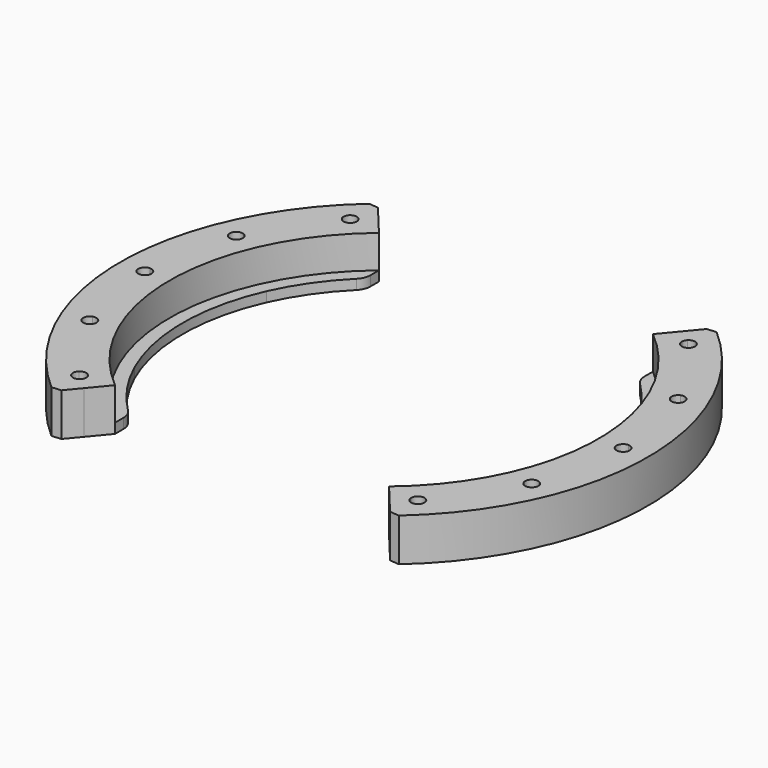
from build123d import *

# Parameters (mm, degrees)
F1_DEPTH    = 3
F2_DEPTH    = 13
F3_R        = 5
F4_T1_DEPTH = 23.5438904605


# Not quite as in the source:
# - a fillet or chamfer that OpenCascade refuses, or shapes differently, is made with other operations: its cross-section is extruded or revolved along the edge and cut away or added


with BuildPart() as f1:
    # F0 (on Top) → F1 (new body)
    with BuildSketch(Plane.XY):
        with BuildLine():
            ThreePointArc((-55.641710973, -25), (-61, 0), (-55.641710973, 25))
            ThreePointArc((-55.641710973, 25), (-49.5734728737, 35.5453342541), (-41.5331193146, 44.6766158074))
            Line((-41.5331193146, 44.6766158074), (-41.5331193146, 50))
            ThreePointArc((-41.5331193146, 50), (-65, 0), (-41.5331193146, -50))
            Line((-41.5331193146, -50), (-41.5331193146, -44.6766158074))
            ThreePointArc((-41.5331193146, -44.6766158074), (-49.5734728737, -35.5453342541), (-55.641710973, -25))
        make_face()
    extrude(amount=F1_DEPTH)



with BuildPart() as f1b:
    # F0 (on Top) → F1, piece 2 (new body)
    with BuildSketch(Plane.XY):
        with BuildLine():
            ThreePointArc((-49.8316562129, 52.6598142712), (-48.1036598795, 54.2428604168), (-46.3254023124, 55.7692307692))
            Line((-46.3254023124, 55.7692307692), (-51.1176853103, 61.5384615385))
            ThreePointArc((-51.1176853103, 61.5384615385), (-80, 0), (-51.1176853103, -61.5384615385))
            Line((-51.1176853103, -61.5384615385), (-46.3254023124, -55.7692307692))
            ThreePointArc((-46.3254023124, -55.7692307692), (-48.1036598795, -54.2428604168), (-49.8316562129, -52.6598142712))
            ThreePointArc((-49.8316562129, -52.6598142712), (-52.6794551984, -52.6794551984), (-52.6598142712, -49.8316562129))
            ThreePointArc((-52.6598142712, -49.8316562129), (-60.2815468919, -40.2788418939), (-66.1904857193, -29.581575351))
            ThreePointArc((-66.1904857193, -29.581575351), (-68.8290251721, -28.5099157112), (-67.721073831, -25.8864087733))
            ThreePointArc((-67.721073831, -25.8864087733), (-71.1069328292, -14.1440483462), (-72.4724137931, -1.9998097412))
            ThreePointArc((-72.4724137931, -1.9998097412), (-74.5, 0), (-72.4724137931, 1.9998097412))
            ThreePointArc((-72.4724137931, 1.9998097412), (-71.1069328292, 14.1440483462), (-67.721073831, 25.8864087733))
            ThreePointArc((-67.721073831, 25.8864087733), (-68.8290251721, 28.5099157112), (-66.1904857193, 29.581575351))
            ThreePointArc((-66.1904857193, 29.581575351), (-60.2815468919, 40.2788418939), (-52.6598142712, 49.8316562129))
            ThreePointArc((-52.6598142712, 49.8316562129), (-52.6794551984, 52.6794551984), (-49.8316562129, 52.6598142712))
        make_face()
    extrude(amount=F1_DEPTH)


with BuildPart() as f1_1:
    add(f1.part)

    add(f1b.part)  # F2 merges F1b
    # F0 (on Top) → F2 (join)
    with BuildSketch(Plane.XY):
        with BuildLine():
            ThreePointArc((-41.5331193146, -50), (-65, 0), (-41.5331193146, 50))
            Line((-41.5331193146, 50), (-46.3254023124, 55.7692307692))
            ThreePointArc((-46.3254023124, 55.7692307692), (-48.1036598795, 54.2428604168), (-49.8316562129, 52.6598142712))
            ThreePointArc((-49.8316562129, 52.6598142712), (-49.4122479979, 52.0178468293), (-49.265241636, 51.265241636))
            ThreePointArc((-49.265241636, 51.265241636), (-50.4871495047, 49.4228050333), (-52.6598142712, 49.8316562129))
            ThreePointArc((-52.6598142712, 49.8316562129), (-60.2815468919, 40.2788418939), (-66.1904857193, 29.581575351))
            ThreePointArc((-66.1904857193, 29.581575351), (-65.3107032116, 28.8441940675), (-64.9812661071, 27.7445488465))
            ThreePointArc((-64.9812661071, 27.7445488465), (-65.8586832477, 26.0893123909), (-67.721073831, 25.8864087733))
            ThreePointArc((-67.721073831, 25.8864087733), (-71.1069328292, 14.1440483462), (-72.4724137931, 1.9998097412))
            ThreePointArc((-72.4724137931, 1.9998097412), (-71.0760666424, 1.4044264997), (-70.5, 0))
            ThreePointArc((-70.5, 0), (-71.0760666424, -1.4044264997), (-72.4724137931, -1.9998097412))
            ThreePointArc((-72.4724137931, -1.9998097412), (-71.1069328292, -14.1440483462), (-67.721073831, -25.8864087733))
            ThreePointArc((-67.721073831, -25.8864087733), (-65.8586832477, -26.0893123909), (-64.9812661071, -27.7445488465))
            ThreePointArc((-64.9812661071, -27.7445488465), (-65.3107032116, -28.8441940675), (-66.1904857193, -29.581575351))
            ThreePointArc((-66.1904857193, -29.581575351), (-60.2815468919, -40.2788418939), (-52.6598142712, -49.8316562129))
            ThreePointArc((-52.6598142712, -49.8316562129), (-50.4871495047, -49.4228050333), (-49.265241636, -51.265241636))
            ThreePointArc((-49.265241636, -51.265241636), (-49.4122479979, -52.0178468293), (-49.8316562129, -52.6598142712))
            ThreePointArc((-49.8316562129, -52.6598142712), (-48.1036598795, -54.2428604168), (-46.3254023124, -55.7692307692))
            Line((-46.3254023124, -55.7692307692), (-41.5331193146, -50))
        make_face()
        with BuildLine():
            ThreePointArc((-49.8316562129, 52.6598142712), (-48.1036598795, 54.2428604168), (-46.3254023124, 55.7692307692))
            Line((-46.3254023124, 55.7692307692), (-51.1176853103, 61.5384615385))
            ThreePointArc((-51.1176853103, 61.5384615385), (-80, 0), (-51.1176853103, -61.5384615385))
            Line((-51.1176853103, -61.5384615385), (-46.3254023124, -55.7692307692))
            ThreePointArc((-46.3254023124, -55.7692307692), (-48.1036598795, -54.2428604168), (-49.8316562129, -52.6598142712))
            ThreePointArc((-49.8316562129, -52.6598142712), (-52.6794551984, -52.6794551984), (-52.6598142712, -49.8316562129))
            ThreePointArc((-52.6598142712, -49.8316562129), (-60.2815468919, -40.2788418939), (-66.1904857193, -29.581575351))
            ThreePointArc((-66.1904857193, -29.581575351), (-68.8290251721, -28.5099157112), (-67.721073831, -25.8864087733))
            ThreePointArc((-67.721073831, -25.8864087733), (-71.1069328292, -14.1440483462), (-72.4724137931, -1.9998097412))
            ThreePointArc((-72.4724137931, -1.9998097412), (-74.5, 0), (-72.4724137931, 1.9998097412))
            ThreePointArc((-72.4724137931, 1.9998097412), (-71.1069328292, 14.1440483462), (-67.721073831, 25.8864087733))
            ThreePointArc((-67.721073831, 25.8864087733), (-68.8290251721, 28.5099157112), (-66.1904857193, 29.581575351))
            ThreePointArc((-66.1904857193, 29.581575351), (-60.2815468919, 40.2788418939), (-52.6598142712, 49.8316562129))
            ThreePointArc((-52.6598142712, 49.8316562129), (-52.6794551984, 52.6794551984), (-49.8316562129, 52.6598142712))
        make_face()
    extrude(amount=F2_DEPTH)

    # F3
    f3_edges = [f1_1.edges().sort_by_distance(p)[0] for p in [
        (-41.533119, 44.676616, 1.5),
        (-41.533119, -44.676616, 1.5),
    ]]
    fillet(f3_edges, radius=F3_R)

    # F4: chamfer of 2 on 2 edges, made by hand

    # F4_s2 → F4_t1 (cut)
    with BuildSketch(Plane.XY.offset(-5.2719452303)):
        with BuildLine():
            Line((-52.6787878448, 60.2075187265), (-49.8233566102, 59.9802728911))
            Line((-49.8233566102, 59.9802728911), (-51.1176853103, 61.5384615385))
            ThreePointArc((-51.1176853103, 61.5384615385), (-51.9240174848, 60.8596451538), (-52.6787878448, 60.2075187265))
        make_face()
        with BuildLine():
            Line((-49.8233566102, -59.9802728911), (-52.6787878448, -60.2075187265))
            ThreePointArc((-52.6787878448, -60.2075187265), (-51.9240174848, -60.8596451538), (-51.1176853103, -61.5384615385))
            Line((-51.1176853103, -61.5384615385), (-49.8233566102, -59.9802728911))
        make_face()
    extrude(amount=F4_T1_DEPTH, mode=Mode.SUBTRACT)


with BuildPart() as f5_1:
    # F5: instance of F1
    add(f1_1.part.mirror(Plane.YZ))


solid = Compound([f1_1.part, f5_1.part])
